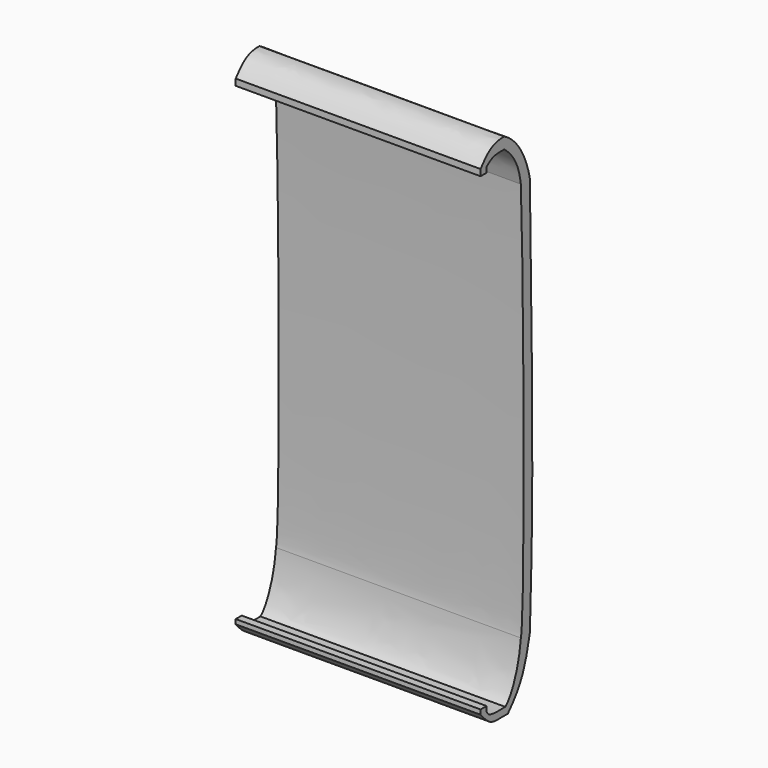
from build123d import *

# Parameters (mm, degrees)
F1_DEPTH = 65


# Not quite as in the source:
# - a feature of the source that left no trace in its solid (it failed there, or was rolled back) is left out


with BuildPart() as f1:
    # F0 (on Right) → F1 (new body)
    with BuildSketch(Plane.YZ):
        with BuildLine():
            add(Edge.make_bspline(
                [(18.7661014497, 0), (19.1870545514, -1.5757839415), (20.9180506756, -1.5757839415), (24.9482551811, -1.4842043442)],
                knots=[0, 0, 0, 0, 6.3578209548, 6.3578209548, 6.3578209548, 6.3578209548], degree=3))
            Line((18.7661014497, 0), (18.7661014497, 1.2257922208))
            Line((18.7661014497, 1.2257922208), (16.7661014497, 1.2257922208))
            Line((16.7661014497, 1.2257922208), (16.7661014497, 0))
            add(Edge.make_bspline(
                [(25.8208457381, -3.4455822315), (20.3640181571, -3.5696015693), (20.0367699781, -3.7762995344), (16.7661014497, 0)],
                knots=[0, 0, 0, 0, 9.6881593216, 9.6881593216, 9.6881593216, 9.6881593216], degree=3))
            add(Edge.make_bspline(
                [(33.1323030144, 12.5043019652), (31.2740066807, 3.1586566474), (29.4667687267, 0.669103465), (25.8208457381, -3.4455822315)],
                knots=[0, 0, 0, 0, 17.5458317954, 17.5458317954, 17.5458317954, 17.5458317954], degree=3))
            add(Edge.make_bspline(
                [(33.1323030144, 118.5604482889), (33.596022293, 83.0767303705), (34.6795393378, 49.8848743737), (33.1323030144, 12.5043019652)],
                knots=[0, 0, 0, 0, 106.0561463237, 106.0561463237, 106.0561463237, 106.0561463237], degree=3))
            add(Edge.make_bspline(
                [(24.665299803, 131.9109736681), (30.0977956504, 129.0076056719), (32.4164180309, 122.3780736327), (33.1323030144, 118.5604482889)],
                knots=[0, 0, 0, 0, 15.8090692731, 15.8090692731, 15.8090692731, 15.8090692731], degree=3))
            add(Edge.make_bspline(
                [(16.7661014497, 127.5289058685), (19.3061102182, 130.8498382568), (21.2166272104, 132.0254335403), (24.665299803, 131.9109736681)],
                knots=[0, 0, 0, 0, 9.0332636862, 9.0332636862, 9.0332636862, 9.0332636862], degree=3))
            Line((16.7661014497, 127.5289058685), (16.7661014497, 125.8308589458))
            Line((16.7661014497, 125.8308589458), (18.7661014497, 125.8308589458))
            Line((18.7661014497, 125.8308589458), (18.7661014497, 127.25))
            add(Edge.make_bspline(
                [(18.7661014497, 127.25), (20.7947045565, 129.0723085403), (22.4061720073, 128.9570778608), (24.665299803, 128.9109736681)],
                knots=[0, 0, 0, 0, 6.1285703665, 6.1285703665, 6.1285703665, 6.1285703665], degree=3))
            add(Edge.make_bspline(
                [(24.665299803, 128.9109736681), (28.353670612, 125.8680671453), (29.4868368655, 122.7559670806), (30.1323030144, 118.5604482889)],
                knots=[0, 0, 0, 0, 11.705618298, 11.705618298, 11.705618298, 11.705618298], degree=3))
            add(Edge.make_bspline(
                [(30.1323030144, 118.5604482889), (31.2795434147, 87.6652374864), (31.466094777, 17.4715379253), (30.1323030144, 12.5043019652)],
                knots=[0, 0, 0, 0, 106.0561463237, 106.0561463237, 106.0561463237, 106.0561463237], degree=3))
            add(Edge.make_bspline(
                [(30.1323030144, 12.5043019652), (29.5598134398, 5.9633483179), (27.0264066677, 0), (24.9482551811, -1.4842043442)],
                knots=[0, 0, 0, 0, 14.9181989766, 14.9181989766, 14.9181989766, 14.9181989766], degree=3))
        make_face()
    extrude(amount=F1_DEPTH)


solid = f1.part
